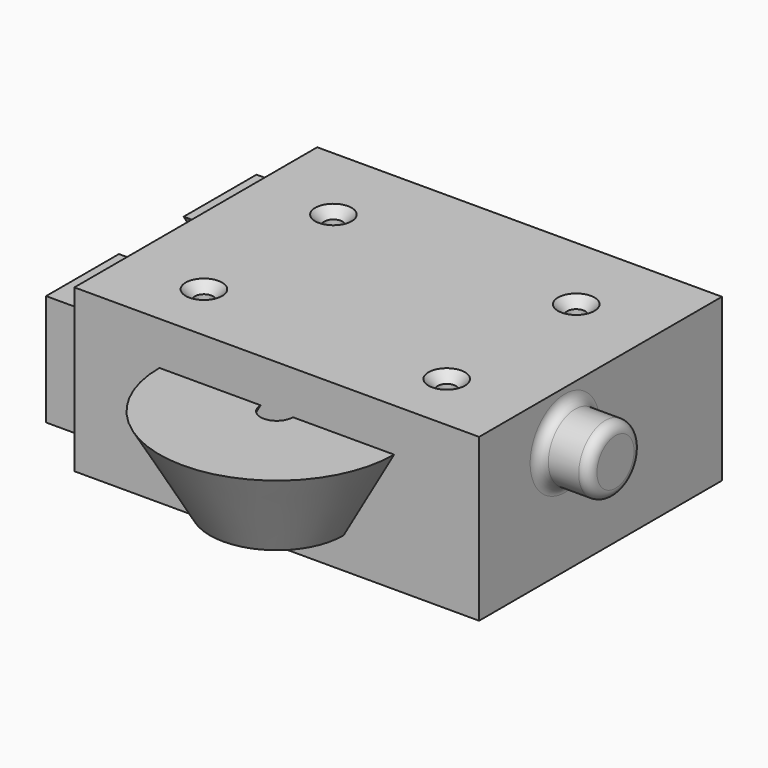
from build123d import *

# Parameters (mm, degrees)
F0_W            = 200
F0_H            = 150
F1_DEPTH        = 80
F13_D           = 9
F13_CSINK_D     = 18
F13_CSINK_ANGLE = 90
F2_R            = 16.4559911856
F3_DEPTH        = 60
F4_DEPTH        = 25
F14_R           = 5
F5_R            = 5
F11_DEPTH       = 22


# Not quite as in the source:
# - a pattern or mirror of a feature is missing from the dataset's text; its kind, count and spacing are read off the source's solid


with BuildPart() as f1:
    # F0 (on Top) → F1 (new body)
    with BuildSketch(Plane.XY):
        Rectangle(F0_W, F0_H)
    extrude(amount=F1_DEPTH)

    # F13 (through all)
    with Locations(Plane.XY.offset(80)):
        with Locations((-60, 35), (-60, -45), (60, 35), (60, -45)):
            CounterSinkHole(F13_D / 2, F13_CSINK_D / 2, counter_sink_angle=F13_CSINK_ANGLE)

    # F2 (on face) → F4 (join)
    with BuildSketch(Plane.YZ.offset(100)):
        with Locations((-21.9944119453, 55.6955486536)):
            Circle(F2_R)
    extrude(amount=F4_DEPTH)

    # F14
    f14_edges = [f1.edges().sort_by_distance(p)[0] for p in [
        (100, -38.450403, 55.695549),
        (125, -38.450403, 55.695549),
    ]]
    fillet(f14_edges, radius=F14_R)

    # F7 (on face) → F15 (revolve)
    with BuildSketch(Plane.XZ.offset(75)):
        Polygon((8, 58.6291704433), (33, 15.327900254), (58, 58.6291704433), align=None)
    revolve(axis=Axis((0, -75, 40), (0, 0, -1)))

    # F10 (on face) → F11 (join)
    with BuildSketch(Plane(origin=(-100, 0, 0), x_dir=(0, -1, 0), z_dir=(-1, 0, 0))):
        Polygon((-20, 65), (-65, 65), (-65, 10), (-20, 10), (-20, 30), (-42.5, 30), align=None)
    f11 = extrude(amount=F11_DEPTH)

    # F11_copies: F11 across plane
    add(f11.mirror(Plane(origin=(0, 0, 0), x_dir=(0, 0, -1), z_dir=(0, -1, 0))))


with BuildPart() as f3:
    # F2 (on face) → F3 (new body)
    with BuildSketch(Plane.YZ.offset(100)):
        with Locations((78.0055880547, 135.6955486536)):
            Circle(F2_R)
    extrude(amount=F3_DEPTH)

    # F5
    f5_edges = [f3.edges().sort_by_distance(p)[0] for p in [
        (160, 61.549597, 135.695549),
        (100, 61.549597, 135.695549),
    ]]
    fillet(f5_edges, radius=F5_R)


with BuildPart() as f6_1:
    # F6: instance of F3
    add(f3.part.mirror(Plane.YZ))


solid = f1.part
